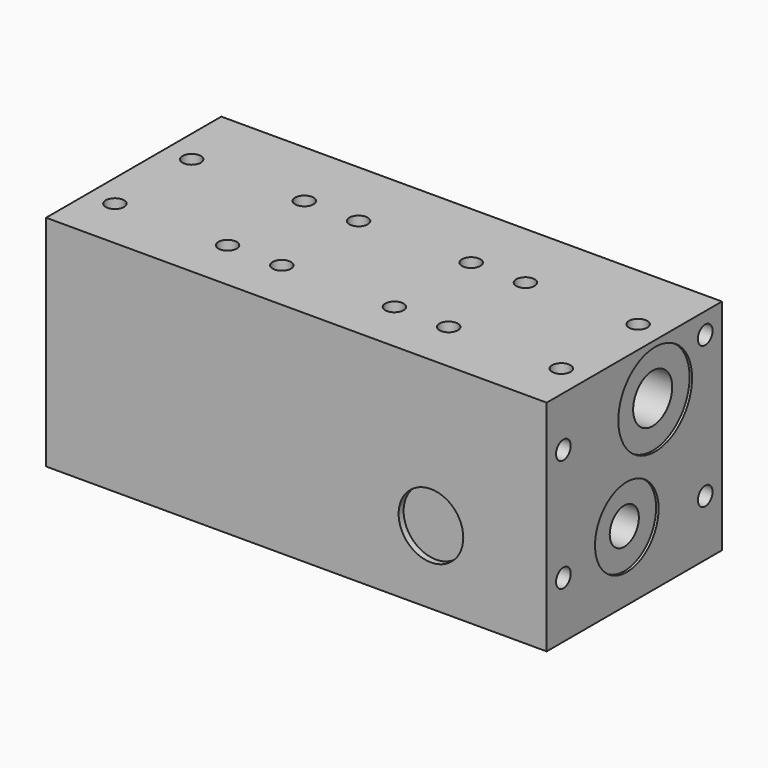
from build123d import *

# Parameters (mm, degrees)
F0_W      = 105
F0_H      = 105
F1_DEPTH  = 240
F3_D      = 8.8
F3_DEPTH  = 20
F3_TIP    = 2.6437867237
F4_D      = 17.4625
F5_D      = 23.41626
F2_R      = 19.05
F2_R_2    = 22.1
F6_DEPTH  = 1.2
F8_D      = 13.49248
F8_DEPTH  = 50
F8_TIP    = 4.0535499425
F7_R      = 14
F9_DEPTH  = 1.2
F11_D     = 8.8
F11_DEPTH = 20
F11_TIP   = 2.6437867237
F13_D     = 8.8
F13_DEPTH = 20
F13_TIP   = 2.6437867237
F14_R     = 15.5
F15_DEPTH = 3


# Not quite as in the source:
# - a feature names something its author has since deleted; it is built from what else it names


with BuildPart() as f1:
    # F0 (on Right) → F1 (new body)
    with BuildSketch(Plane.YZ):
        Rectangle(F0_W, F0_H)
    extrude(amount=F1_DEPTH)

    # F3
    with Locations(Plane.YZ.offset(240)):
        with Locations((-42.5, 28.5), (42.5, 42.5), (42.5, -25.5), (-42.5, -25.5)):
            Hole(F3_D / 2, depth=F3_DEPTH)
            with Locations((0, 0, -(F3_DEPTH + F3_TIP / 2))):  # 118° drill point
                Cone(0, F3_D / 2, F3_TIP, mode=Mode.SUBTRACT)

    # F4 (through all)
    with Locations(Plane.YZ.offset(240)):
        with Locations((-4.5, -19.5)):
            Hole(F4_D / 2)

    # F5 (through all)
    with Locations(Plane.YZ.offset(240)):
        with Locations((12.5, 27.5)):
            Hole(F5_D / 2)

    # F2 (on face) → F6 (cut)
    with BuildSketch(Plane.YZ.offset(240)):
        with Locations((-4.5, -19.5)):
            Circle(F2_R)
        with Locations((12.5, 27.5)):
            Circle(F2_R_2)
    extrude(amount=-F6_DEPTH, mode=Mode.SUBTRACT)

    # F8
    with Locations(Plane(origin=(0, 52.5, 0), x_dir=(-1, 0, 0), z_dir=(0, 1, 0))):
        with Locations((-200, 27.5), (-200, -32.5), (-120, -32.5), (-120, 27.5), (-40, 27.5), (-40, -32.5), (40, -32.5), (40, 27.5), (120, 27.5), (120, -32.5), (200, -32.5), (200, 27.5), (280, 27.5), (280, -32.5)):
            Hole(F8_D / 2, depth=F8_DEPTH)
            with Locations((0, 0, -(F8_DEPTH + F8_TIP / 2))):  # 118° drill point
                Cone(0, F8_D / 2, F8_TIP, mode=Mode.SUBTRACT)

    # F7 (on face) → F9 (cut)
    with BuildSketch(Plane(origin=(0, 52.5, 0), x_dir=(-1, 0, 0), z_dir=(0, 1, 0))):
        with Locations((-200, 27.5)):
            Circle(F7_R)
        with Locations((-200, -32.5)):
            Circle(F7_R)
        with Locations((-120, 27.5)):
            Circle(F7_R)
        with Locations((-120, -32.5)):
            Circle(F7_R)
        with Locations((-40, 27.5)):
            Circle(F7_R)
        with Locations((-40, -32.5)):
            Circle(F7_R)
        with Locations((40, 27.5)):
            Circle(F7_R)
        with Locations((40, -32.5)):
            Circle(F7_R)
        with Locations((120, 27.5)):
            Circle(F7_R)
        with Locations((120, -32.5)):
            Circle(F7_R)
        with Locations((200, 27.5)):
            Circle(F7_R)
        with Locations((200, -32.5)):
            Circle(F7_R)
        with Locations((280, 27.5)):
            Circle(F7_R)
        with Locations((280, -32.5)):
            Circle(F7_R)
    extrude(amount=-F9_DEPTH, mode=Mode.SUBTRACT)

    # F11
    with Locations(Plane.XY.offset(52.5)):
        with Locations((13, 18.5), (13, -27.5), (67, -27.5), (67, 18.5), (93, 18.5), (93, -27.5), (147, 18.5), (147, -27.5), (173, -27.5), (173, 18.5), (227, 18.5), (227, -27.5)):
            Hole(F11_D / 2, depth=F11_DEPTH)
            with Locations((0, 0, -(F11_DEPTH + F11_TIP / 2))):  # 118° drill point
                Cone(0, F11_D / 2, F11_TIP, mode=Mode.SUBTRACT)

    # F13
    with Locations(Plane(origin=(0, 0, -52.5), x_dir=(1, 0, 0), z_dir=(0, 0, -1))):
        with Locations((12, 40.5), (12, -40.5), (228, -40.5), (228, 40.5)):
            Hole(F13_D / 2, depth=F13_DEPTH)
            with Locations((0, 0, -(F13_DEPTH + F13_TIP / 2))):  # 118° drill point
                Cone(0, F13_D / 2, F13_TIP, mode=Mode.SUBTRACT)

    # F14 (on face) → F15 (cut)
    with BuildSketch(Plane.XZ.offset(52.5)):
        with Locations((184.5, -17.5)):
            Circle(F14_R)
    extrude(amount=-F15_DEPTH, mode=Mode.SUBTRACT)


solid = f1.part
